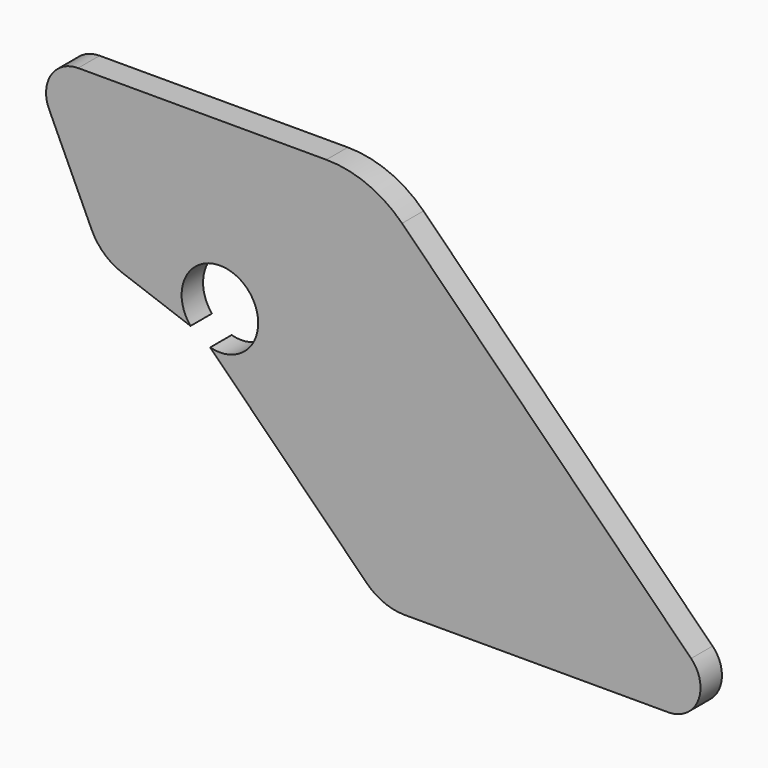
from build123d import *

# Parameters (mm, degrees)
F1_DEPTH = 25


# Not quite as in the source:
# - ends of sketch curves that miss each other by under 0.0002 mm in the source are joined


with BuildPart() as f1:
    # F0 (on Front) → F1 (new body)
    with BuildSketch(Plane.XZ):
        with BuildLine():
            ThreePointArc((-170.642238, -2.693902), (-124.029000476, 50.3717259287), (-152.294215, -14.357189))
            Line((-152.294215, -14.357189), (-6.118396, -160.533008))
            ThreePointArc((-6.118396, -160.533008), (10.1027713817, -171.3716456256), (29.236943, -175.177669))
            Line((29.236943, -175.177669), (275.511113, -175.177669))
            ThreePointArc((275.511113, -175.177669), (303.22749884, -156.6581722976), (296.7243169356, -123.9644660644))
            Line((296.7243169356, -123.9644660644), (26.871503, 145.888348))
            ThreePointArc((26.871503, 145.888348), (-5.5708317635, 167.5656232511), (-43.839175, 175.17767))
            Line((-43.839175, 175.17767), (-275.511114, 175.17767))
            ThreePointArc((-275.511114, 175.17767), (-300.7842187682, 161.3415239766), (-302.7451656672, 132.5956816918))
            Line((-302.7451656672, 132.5956816918), (-262.960739, 46.481221))
            ThreePointArc((-262.960739, 46.481221), (-251.37881686, 30.6136107366), (-234.5779690393, 20.4325748914))
            Line((-234.5779690393, 20.4325748914), (-170.642238, -2.693902))
        make_face()
    extrude(amount=F1_DEPTH)


solid = f1.part
